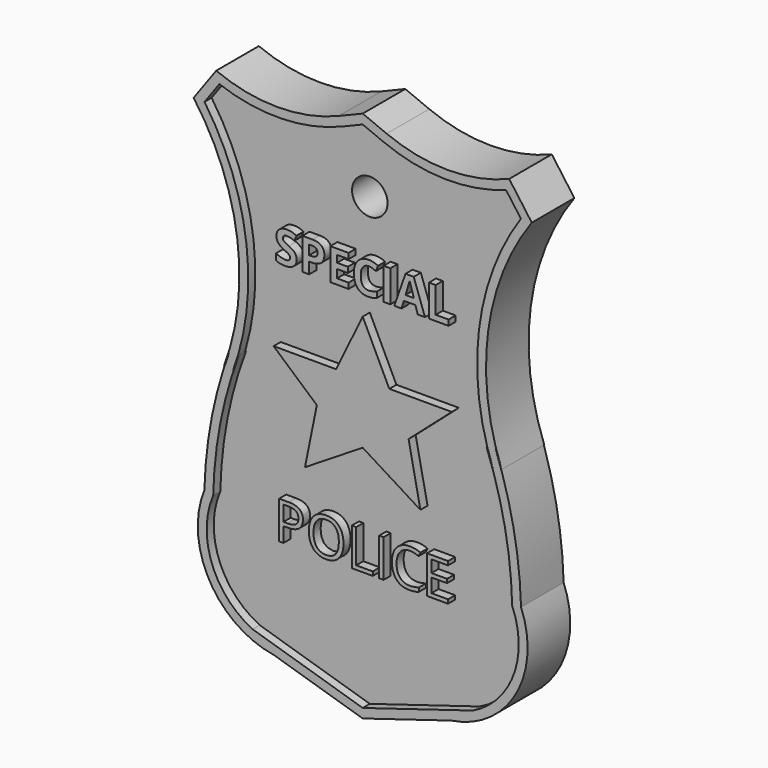
from build123d import *

# Parameters (mm, degrees)
F0_W           = 0.4923276621
F0_H           = 4.2362431042
F0_R           = 2
F0_W_2         = 0.7584236685
F0_H_2         = 3.5760967401
F1_DEPTH       = 5
F0_TEXT_SIZE   = 5.0091965718
F0_TEXT_SIZE_2 = 5.9338927263
F2_DEPTH       = 6


# Not quite as in the source:
# - a feature names something its author has since deleted; it is built from what else it names
# - Text() gives the source's letters only with a copy of the font that has no kerning and outlines rounded to 1/6400 em; it was checked with that copy


with BuildPart() as f1:
    # F0 (on Front) → F1 (new body)
    with BuildSketch(Plane.XZ):
        with BuildLine():
            Line((2.6978656745, 27.0723157725), (0, 28.1849289482))
            Line((0, 28.1849289482), (-2.6978656745, 27.0723157725))
            ThreePointArc((-2.6978656745, 27.0723157725), (-9.601713641, 25.7045974419), (-16.5055616074, 27.0723157725))
            Line((-16.5055616074, 27.0723157725), (-19.0506021551, 23.561483789))
            ThreePointArc((-19.0506021551, 23.561483789), (-14.1307840894, 11.1964219838), (-15.6559578137, -2.0237598742))
            Line((-15.6559578137, -2.0237598742), (-14.8904452178, 0))
            ThreePointArc((-14.8904452178, 0), (-16.9912920381, -7.3586022254), (-17.8392625093, -14.9640956448))
            ThreePointArc((-17.8392625093, -14.9640956448), (-17.2572372048, -23.7734712257), (-9.9838551694, -28.7776460174))
            Line((-9.9838551694, -28.7776460174), (0, -31.8150710518))
            Line((0, -31.8150710518), (9.9838551694, -28.7776460174))
            ThreePointArc((9.9838551694, -28.7776460174), (17.2572372048, -23.7734712257), (17.8392625093, -14.9640956448))
            ThreePointArc((17.8392625093, -14.9640956448), (16.9912920381, -7.3586022254), (14.8904452178, 0))
            Line((14.8904452178, 0), (15.6559578137, -2.0237598742))
            ThreePointArc((15.6559578137, -2.0237598742), (14.1307840894, 11.1964219838), (19.0506021551, 23.561483789))
            Line((19.0506021551, 23.561483789), (16.5055616074, 27.0723157725))
            ThreePointArc((16.5055616074, 27.0723157725), (9.601713641, 25.7045974419), (2.6978656745, 27.0723157725))
        make_face()
        with BuildLine():
            Line((-17.8220764571, 23.5524013394), (-16.1484710633, 25.8611061456))
            ThreePointArc((-16.1484710633, 25.8611061456), (-9.2056785313, 24.7087019846), (-2.3166098411, 26.1478462006))
            Line((-2.3166098411, 26.1478462006), (0, 27.1032275809))
            Line((0, 27.1032275809), (2.3166098411, 26.1478462006))
            ThreePointArc((2.3166098411, 26.1478462006), (9.2056785313, 24.7087019846), (16.1484710633, 25.8611061456))
            Line((16.1484710633, 25.8611061456), (17.8220764571, 23.5524013394))
            ThreePointArc((17.8220764571, 23.5524013394), (13.0939999284, 10.9674605371), (14.7206357065, -2.3775572112))
            Line((14.7206357065, -2.3775572112), (13.9551231106, -0.353797337))
            ThreePointArc((13.9551231106, -0.353797337), (16.0279163768, -7.642539104), (16.8443387914, -15.1761758693))
            ThreePointArc((16.8443387914, -15.1761758693), (16.9968634432, -21.9803415725), (12.3984711461, -26.9977834474))
            Line((12.3984711461, -26.9977834474), (0, -30.7698159948))
            Line((0, -30.7698159948), (-12.3984711461, -26.9977834474))
            ThreePointArc((-12.3984711461, -26.9977834474), (-16.9968634432, -21.9803415725), (-16.8443387914, -15.1761758693))
            ThreePointArc((-16.8443387914, -15.1761758693), (-16.0279163768, -7.642539104), (-13.9551231106, -0.353797337))
            Line((-13.9551231106, -0.353797337), (-14.7206357065, -2.3775572112))
            ThreePointArc((-14.7206357065, -2.3775572112), (-13.0939999284, 10.9674605371), (-17.8220764571, 23.5524013394))
        make_face(mode=Mode.SUBTRACT)
        with BuildLine():
            ThreePointArc((-2.3166098411, 26.1478462006), (-9.2056785313, 24.7087019846), (-16.1484710633, 25.8611061456))
            Line((-16.1484710633, 25.8611061456), (-17.8220764571, 23.5524013394))
            ThreePointArc((-17.8220764571, 23.5524013394), (-13.0939999284, 10.9674605371), (-14.7206357065, -2.3775572112))
            Line((-14.7206357065, -2.3775572112), (-13.9551231106, -0.353797337))
            ThreePointArc((-13.9551231106, -0.353797337), (-16.0279163768, -7.642539104), (-16.8443387914, -15.1761758693))
            ThreePointArc((-16.8443387914, -15.1761758693), (-16.9968634432, -21.9803415725), (-12.3984711461, -26.9977834474))
            Line((-12.3984711461, -26.9977834474), (0, -30.7698159948))
            Line((0, -30.7698159948), (12.3984711461, -26.9977834474))
            ThreePointArc((12.3984711461, -26.9977834474), (16.9968634432, -21.9803415725), (16.8443387914, -15.1761758693))
            ThreePointArc((16.8443387914, -15.1761758693), (16.0279163768, -7.642539104), (13.9551231106, -0.353797337))
            Line((13.9551231106, -0.353797337), (14.7206357065, -2.3775572112))
            ThreePointArc((14.7206357065, -2.3775572112), (13.0939999284, 10.9674605371), (17.8220764571, 23.5524013394))
            Line((17.8220764571, 23.5524013394), (16.1484710633, 25.8611061456))
            ThreePointArc((16.1484710633, 25.8611061456), (9.2056785313, 24.7087019846), (2.3166098411, 26.1478462006))
            Line((2.3166098411, 26.1478462006), (0, 27.1032275809))
            Line((0, 27.1032275809), (-2.3166098411, 26.1478462006))
        make_face()
        with BuildLine():
            add(Edge.make_bspline(
                [(-8.3190394511, -13.0703245643), (-6.7317231468, -13.0703245643), (-6.7317231468, -14.3043888173)],
                knots=[0, 0, 0, 1, 1, 1], degree=2))
            add(Edge.make_bspline(
                [(-6.7317231468, -14.3043888173), (-6.7317231468, -14.9478453098), (-7.1707384915, -15.2941435806)],
                knots=[0, 0, 0, 1, 1, 1], degree=2))
            add(Edge.make_bspline(
                [(-7.1707384915, -15.2941435806), (-7.6097538362, -15.6404418514), (-8.4265912568, -15.6404418514)],
                knots=[0, 0, 0, 1, 1, 1], degree=2))
            Line((-8.4265912568, -15.6404418514), (-8.9254091141, -15.6404418514))
            Line((-8.9254091141, -15.6404418514), (-8.9254091141, -17.3065676685))
            Line((-8.9254091141, -17.3065676685), (-9.4177367762, -17.3065676685))
            Line((-9.4177367762, -17.3065676685), (-9.4177367762, -13.0703245643))
            Line((-9.4177367762, -13.0703245643), (-8.3190394511, -13.0703245643))
        make_face(mode=Mode.SUBTRACT)
        with BuildLine():
            add(Edge.make_bspline(
                [(-2.6809141903, -13.5830499827), (-2.168188772, -14.1625316943), (-2.168188772, -15.1824195066)],
                knots=[0, 0, 0, 1, 1, 1], degree=2))
            add(Edge.make_bspline(
                [(-2.168188772, -15.1824195066), (-2.168188772, -16.1995258068), (-2.6827685318, -16.7822526159)],
                knots=[0, 0, 0, 1, 1, 1], degree=2))
            add(Edge.make_bspline(
                [(-2.6827685318, -16.7822526159), (-3.1973482917, -17.364979425), (-4.1124658106, -17.364979425)],
                knots=[0, 0, 0, 1, 1, 1], degree=2))
            add(Edge.make_bspline(
                [(-4.1124658106, -17.364979425), (-5.0479810857, -17.364979425), (-5.5565342358, -16.792451494)],
                knots=[0, 0, 0, 1, 1, 1], degree=2))
            add(Edge.make_bspline(
                [(-5.5565342358, -16.792451494), (-6.0650873858, -16.219923563), (-6.0650873858, -15.1768564822)],
                knots=[0, 0, 0, 1, 1, 1], degree=2))
            add(Edge.make_bspline(
                [(-6.0650873858, -15.1768564822), (-6.0650873858, -14.142133938), (-5.5551434797, -13.5728511046)],
                knots=[0, 0, 0, 1, 1, 1], degree=2))
            add(Edge.make_bspline(
                [(-5.5551434797, -13.5728511046), (-5.0451995735, -13.0035682712), (-4.1069027861, -13.0035682712)],
                knots=[0, 0, 0, 1, 1, 1], degree=2))
            add(Edge.make_bspline(
                [(-4.1069027861, -13.0035682712), (-3.1936396087, -13.0035682712), (-2.6809141903, -13.5830499827)],
                knots=[0, 0, 0, 1, 1, 1], degree=2))
        make_face(mode=Mode.SUBTRACT)
        Polygon((1.1371749108, -17.3065676685), (-1.2243289602, -17.3065676685), (-1.2243289602, -13.0703245643), (-0.732001298, -13.0703245643), (-0.732001298, -16.8605985433), (1.1371749108, -16.8605985433), align=None, mode=Mode.SUBTRACT)
        with Locations((2.1018960642, -15.1884461164)):
            Rectangle(F0_W, F0_H, mode=Mode.SUBTRACT)
        with BuildLine():
            add(Edge.make_bspline(
                [(6.2857540216, -13.6757670566), (5.8045524083, -13.4504645671), (5.323350795, -13.4504645671)],
                knots=[0, 0, 0, 1, 1, 1], degree=2))
            add(Edge.make_bspline(
                [(5.323350795, -13.4504645671), (4.625191229, -13.4504645671), (4.220944787, -13.9154406925)],
                knots=[0, 0, 0, 1, 1, 1], degree=2))
            add(Edge.make_bspline(
                [(4.220944787, -13.9154406925), (3.816698345, -14.3804168178), (3.816698345, -15.1889097018)],
                knots=[0, 0, 0, 1, 1, 1], degree=2))
            add(Edge.make_bspline(
                [(3.816698345, -15.1889097018), (3.816698345, -16.0196546835), (4.2065736405, -16.47350476)],
                knots=[0, 0, 0, 1, 1, 1], degree=2))
            add(Edge.make_bspline(
                [(4.2065736405, -16.47350476), (4.5964489361, -16.9273548365), (5.3177877706, -16.9273548365)],
                knots=[0, 0, 0, 1, 1, 1], degree=2))
            add(Edge.make_bspline(
                [(5.3177877706, -16.9273548365), (5.7609753836, -16.9273548365), (6.3293310463, -16.7678814695)],
                knots=[0, 0, 0, 1, 1, 1], degree=2))
            Line((6.3293310463, -16.7678814695), (6.3293310463, -17.1990158629))
            add(Edge.make_bspline(
                [(6.3293310463, -17.1990158629), (5.8889249455, -17.364979425), (5.2426869408, -17.364979425)],
                knots=[0, 0, 0, 1, 1, 1], degree=2))
            add(Edge.make_bspline(
                [(5.2426869408, -17.364979425), (4.3071716657, -17.364979425), (3.7986185156, -16.7966237623)],
                knots=[0, 0, 0, 1, 1, 1], degree=2))
            add(Edge.make_bspline(
                [(3.7986185156, -16.7966237623), (3.2900653655, -16.2282680997), (3.2900653655, -15.1824195066)],
                knots=[0, 0, 0, 1, 1, 1], degree=2))
            add(Edge.make_bspline(
                [(3.2900653655, -15.1824195066), (3.2900653655, -14.5278369653), (3.5348384405, -14.0355093031)],
                knots=[0, 0, 0, 1, 1, 1], degree=2))
            add(Edge.make_bspline(
                [(3.5348384405, -14.0355093031), (3.7796115155, -13.543181641), (4.2418061286, -13.2766200537)],
                knots=[0, 0, 0, 1, 1, 1], degree=2))
            add(Edge.make_bspline(
                [(4.2418061286, -13.2766200537), (4.7040007417, -13.0100584663), (5.3298409902, -13.0100584663)],
                knots=[0, 0, 0, 1, 1, 1], degree=2))
            add(Edge.make_bspline(
                [(5.3298409902, -13.0100584663), (5.9955495805, -13.0100584663), (6.4943674378, -13.2529771998)],
                knots=[0, 0, 0, 1, 1, 1], degree=2))
            Line((6.4943674378, -13.2529771998), (6.2857540216, -13.6757670566))
        make_face(mode=Mode.SUBTRACT)
        Polygon((9.6152241435, -16.8661615677), (9.6152241435, -17.3065676685), (7.2537202726, -17.3065676685), (7.2537202726, -13.0703245643), (9.6152241435, -13.0703245643), (9.6152241435, -13.5079491529), (7.7460479347, -13.5079491529), (7.7460479347, -14.87274448), (9.5021093134, -14.87274448), (9.5021093134, -15.3075875563), (7.7460479347, -15.3075875563), (7.7460479347, -16.8661615677), align=None, mode=Mode.SUBTRACT)
        Polygon((-2.9973116953, 1.8562454497), (0, 8.0466551414), (2.9973116953, 1.8562454497), (10.0362910237, 1.8562454497), (5.1685351705, -2.4151530963), (6.5026363504, -9.0073454569), (0, -4.953042775), (-6.5026363504, -9.0073454569), (-5.1685351705, -2.4151530963), (-10.0362910237, 1.8562454497), align=None, mode=Mode.SUBTRACT)
        with BuildLine():
            add(Edge.make_bspline(
                [(-7.6249364067, 11.858161132), (-7.4390482527, 11.6174848904), (-7.4390482527, 11.2676238174)],
                knots=[0, 0, 0, 1, 1, 1], degree=2))
            add(Edge.make_bspline(
                [(-7.4390482527, 11.2676238174), (-7.4390482527, 10.7831405864), (-7.7877352953, 10.5041126836)],
                knots=[0, 0, 0, 1, 1, 1], degree=2))
            add(Edge.make_bspline(
                [(-7.7877352953, 10.5041126836), (-8.1364223379, 10.2250847809), (-8.7570931006, 10.2250847809)],
                knots=[0, 0, 0, 1, 1, 1], degree=2))
            add(Edge.make_bspline(
                [(-8.7570931006, 10.2250847809), (-9.3300199585, 10.2250847809), (-9.7698900325, 10.441106383)],
                knots=[0, 0, 0, 1, 1, 1], degree=2))
            Line((-9.7698900325, 10.441106383), (-9.7698900325, 11.1455246509))
            add(Edge.make_bspline(
                [(-9.7698900325, 11.1455246509), (-9.408288655, 10.9835084493), (-9.1574374829, 10.9177627443)],
                knots=[0, 0, 0, 1, 1, 1], degree=2))
            add(Edge.make_bspline(
                [(-9.1574374829, 10.9177627443), (-8.9065863108, 10.8520170393), (-8.6983915783, 10.8520170393)],
                knots=[0, 0, 0, 1, 1, 1], degree=2))
            add(Edge.make_bspline(
                [(-8.6983915783, 10.8520170393), (-8.4494971236, 10.8520170393), (-8.3160489962, 10.9471135055)],
                knots=[0, 0, 0, 1, 1, 1], degree=2))
            add(Edge.make_bspline(
                [(-8.3160489962, 10.9471135055), (-8.1826008688, 11.0422099716), (-8.1826008688, 11.23083753)],
                knots=[0, 0, 0, 1, 1, 1], degree=2))
            add(Edge.make_bspline(
                [(-8.1826008688, 11.23083753), (-8.1826008688, 11.3357175833), (-8.2413023911, 11.4178997145)],
                knots=[0, 0, 0, 1, 1, 1], degree=2))
            add(Edge.make_bspline(
                [(-8.2413023911, 11.4178997145), (-8.3000039134, 11.5000818458), (-8.4138848667, 11.5756111378)],
                knots=[0, 0, 0, 1, 1, 1], degree=2))
            add(Edge.make_bspline(
                [(-8.4138848667, 11.5756111378), (-8.5277658201, 11.6511404299), (-8.8776268931, 11.8178527533)],
                knots=[0, 0, 0, 1, 1, 1], degree=2))
            add(Edge.make_bspline(
                [(-8.8776268931, 11.8178527533), (-9.2047900442, 11.9720420853), (-9.3687629633, 12.1137084258)],
                knots=[0, 0, 0, 1, 1, 1], degree=2))
            add(Edge.make_bspline(
                [(-9.3687629633, 12.1137084258), (-9.5327358823, 12.2553747664), (-9.6305717528, 12.4440023248)],
                knots=[0, 0, 0, 1, 1, 1], degree=2))
            add(Edge.make_bspline(
                [(-9.6305717528, 12.4440023248), (-9.7284076234, 12.6326298832), (-9.7284076234, 12.8838723987)],
                knots=[0, 0, 0, 1, 1, 1], degree=2))
            add(Edge.make_bspline(
                [(-9.7284076234, 12.8838723987), (-9.7284076234, 13.3589633861), (-9.406723281, 13.6301644192)],
                knots=[0, 0, 0, 1, 1, 1], degree=2))
            add(Edge.make_bspline(
                [(-9.406723281, 13.6301644192), (-9.0850389387, 13.9013654524), (-8.5175908895, 13.9013654524)],
                knots=[0, 0, 0, 1, 1, 1], degree=2))
            add(Edge.make_bspline(
                [(-8.5175908895, 13.9013654524), (-8.2389543302, 13.9013654524), (-7.9857550972, 13.8356197474)],
                knots=[0, 0, 0, 1, 1, 1], degree=2))
            add(Edge.make_bspline(
                [(-7.9857550972, 13.8356197474), (-7.7325558643, 13.7698740424), (-7.4562673659, 13.6501229368)],
                knots=[0, 0, 0, 1, 1, 1], degree=2))
            Line((-7.4562673659, 13.6501229368), (-7.7004656987, 13.0599769657))
            add(Edge.make_bspline(
                [(-7.7004656987, 13.0599769657), (-7.9869291277, 13.1773800104), (-8.1739913122, 13.2239498848)],
                knots=[0, 0, 0, 1, 1, 1], degree=2))
            add(Edge.make_bspline(
                [(-8.1739913122, 13.2239498848), (-8.3610534967, 13.2705197591), (-8.5418541854, 13.2705197591)],
                knots=[0, 0, 0, 1, 1, 1], degree=2))
            add(Edge.make_bspline(
                [(-8.5418541854, 13.2705197591), (-8.7570931006, 13.2705197591), (-8.8721480844, 13.1703358277)],
                knots=[0, 0, 0, 1, 1, 1], degree=2))
            add(Edge.make_bspline(
                [(-8.8721480844, 13.1703358277), (-8.9872030681, 13.0701518963), (-8.9872030681, 12.9089183816)],
                knots=[0, 0, 0, 1, 1, 1], degree=2))
            add(Edge.make_bspline(
                [(-8.9872030681, 12.9089183816), (-8.9872030681, 12.8087344502), (-8.9406331938, 12.7339878451)],
                knots=[0, 0, 0, 1, 1, 1], degree=2))
            add(Edge.make_bspline(
                [(-8.9406331938, 12.7339878451), (-8.8940633194, 12.65924124), (-8.7927053575, 12.5895821001)],
                knots=[0, 0, 0, 1, 1, 1], degree=2))
            add(Edge.make_bspline(
                [(-8.7927053575, 12.5895821001), (-8.6913473956, 12.5199229603), (-8.3125269049, 12.3391222716)],
                knots=[0, 0, 0, 1, 1, 1], degree=2))
            add(Edge.make_bspline(
                [(-8.3125269049, 12.3391222716), (-7.8108245607, 12.0988373735), (-7.6249364067, 11.858161132)],
                knots=[0, 0, 0, 1, 1, 1], degree=2))
        make_face(mode=Mode.SUBTRACT)
        with BuildLine():
            add(Edge.make_bspline(
                [(-4.6593354988, 13.5702888665), (-4.3208233867, 13.2900869332), (-4.3208233867, 12.7351618755)],
                knots=[0, 0, 0, 1, 1, 1], degree=2))
            add(Edge.make_bspline(
                [(-4.3208233867, 12.7351618755), (-4.3208233867, 12.1575388958), (-4.6816420773, 11.8518996362)],
                knots=[0, 0, 0, 1, 1, 1], degree=2))
            add(Edge.make_bspline(
                [(-4.6816420773, 11.8518996362), (-5.0424607678, 11.5462603767), (-5.7077446875, 11.5462603767)],
                knots=[0, 0, 0, 1, 1, 1], degree=2))
            Line((-5.7077446875, 11.5462603767), (-6.0325597777, 11.5462603767))
            Line((-6.0325597777, 11.5462603767), (-6.0325597777, 10.2743940596))
            Line((-6.0325597777, 10.2743940596), (-6.7909834462, 10.2743940596))
            Line((-6.7909834462, 10.2743940596), (-6.7909834462, 13.8504907997))
            Line((-6.7909834462, 13.8504907997), (-5.6490431652, 13.8504907997))
            add(Edge.make_bspline(
                [(-5.6490431652, 13.8504907997), (-4.9978476108, 13.8504907997), (-4.6593354988, 13.5702888665)],
                knots=[0, 0, 0, 1, 1, 1], degree=2))
        make_face(mode=Mode.SUBTRACT)
        Polygon((-1.5861151333, 10.9005436311), (-1.5861151333, 10.2743940596), (-3.6453645365, 10.2743940596), (-3.6453645365, 13.8504907997), (-1.5861151333, 13.8504907997), (-1.5861151333, 13.22903735), (-2.886940868, 13.22903735), (-2.886940868, 12.4440023248), (-1.6761241342, 12.4440023248), (-1.6761241342, 11.8225488751), (-2.886940868, 11.8225488751), (-2.886940868, 10.9005436311), align=None, mode=Mode.SUBTRACT)
        with Locations((0, 19.5384901017)):
            Circle(F0_R, mode=Mode.SUBTRACT)
        with BuildLine():
            add(Edge.make_bspline(
                [(1.0773686064, 13.1996865889), (0.8746526827, 13.2705197591), (0.6789809416, 13.2705197591)],
                knots=[0, 0, 0, 1, 1, 1], degree=2))
            add(Edge.make_bspline(
                [(0.6789809416, 13.2705197591), (0.2508511721, 13.2705197591), (0.0160450828, 12.9488354168)],
                knots=[0, 0, 0, 1, 1, 1], degree=2))
            add(Edge.make_bspline(
                [(0.0160450828, 12.9488354168), (-0.2187610065, 12.6271510744), (-0.2187610065, 12.0526588426)],
                knots=[0, 0, 0, 1, 1, 1], degree=2))
            add(Edge.make_bspline(
                [(-0.2187610065, 12.0526588426), (-0.2187610065, 10.8567131611), (0.6789809416, 10.8567131611)],
                knots=[0, 0, 0, 1, 1, 1], degree=2))
            add(Edge.make_bspline(
                [(0.6789809416, 10.8567131611), (1.0554533714, 10.8567131611), (1.590811255, 11.0445580325)],
                knots=[0, 0, 0, 1, 1, 1], degree=2))
            Line((1.590811255, 11.0445580325), (1.590811255, 10.4090162175))
            add(Edge.make_bspline(
                [(1.590811255, 10.4090162175), (1.1509411811, 10.2250847809), (0.6077564278, 10.2250847809)],
                knots=[0, 0, 0, 1, 1, 1], degree=2))
            add(Edge.make_bspline(
                [(0.6077564278, 10.2250847809), (-0.1725824756, 10.2250847809), (-0.5858411928, 10.6986103943)],
                knots=[0, 0, 0, 1, 1, 1], degree=2))
            add(Edge.make_bspline(
                [(-0.5858411928, 10.6986103943), (-0.99909991, 11.1721360077), (-0.99909991, 12.0573549644)],
                knots=[0, 0, 0, 1, 1, 1], degree=2))
            add(Edge.make_bspline(
                [(-0.99909991, 12.0573549644), (-0.99909991, 12.61541077), (-0.7959926427, 13.0349309829)],
                knots=[0, 0, 0, 1, 1, 1], degree=2))
            add(Edge.make_bspline(
                [(-0.7959926427, 13.0349309829), (-0.5928853755, 13.4544511958), (-0.2124995108, 13.6779083241)],
                knots=[0, 0, 0, 1, 1, 1], degree=2))
            add(Edge.make_bspline(
                [(-0.2124995108, 13.6779083241), (0.1678863539, 13.9013654524), (0.6789809416, 13.9013654524)],
                knots=[0, 0, 0, 1, 1, 1], degree=2))
            add(Edge.make_bspline(
                [(0.6789809416, 13.9013654524), (1.1994677729, 13.9013654524), (1.7254334129, 13.6501229368)],
                knots=[0, 0, 0, 1, 1, 1], degree=2))
            Line((1.7254334129, 13.6501229368), (1.48123508, 13.0333656089))
            add(Edge.make_bspline(
                [(1.48123508, 13.0333656089), (1.2800845302, 13.1288534186), (1.0773686064, 13.1996865889)],
                knots=[0, 0, 0, 1, 1, 1], degree=2))
        make_face(mode=Mode.SUBTRACT)
        with Locations((2.7307948186, 12.0624424297)):
            Rectangle(F0_W_2, F0_H_2, mode=Mode.SUBTRACT)
        Polygon((7.0163972919, 10.2743940596), (6.1992721011, 10.2743940596), (5.9402027159, 11.1259574768), (4.6362462333, 11.1259574768), (4.3771768481, 10.2743940596), (3.5600516573, 10.2743940596), (4.8225257308, 13.865361852), (5.7492270966, 13.865361852), align=None, mode=Mode.SUBTRACT)
        Polygon((9.6751849098, 10.2743940596), (7.4664422964, 10.2743940596), (7.4664422964, 13.8504907997), (8.2248659649, 13.8504907997), (8.2248659649, 10.9005436311), (9.6751849098, 10.9005436311), align=None, mode=Mode.SUBTRACT)
    extrude(amount=F1_DEPTH)

    # F0 (on Front) → F2 (join)
    with BuildSketch(Plane.XZ):
        with BuildLine():
            Line((2.6978656745, 27.0723157725), (0, 28.1849289482))
            Line((0, 28.1849289482), (-2.6978656745, 27.0723157725))
            ThreePointArc((-2.6978656745, 27.0723157725), (-9.601713641, 25.7045974419), (-16.5055616074, 27.0723157725))
            Line((-16.5055616074, 27.0723157725), (-19.0506021551, 23.561483789))
            ThreePointArc((-19.0506021551, 23.561483789), (-14.1307840894, 11.1964219838), (-15.6559578137, -2.0237598742))
            Line((-15.6559578137, -2.0237598742), (-14.8904452178, 0))
            ThreePointArc((-14.8904452178, 0), (-16.9912920381, -7.3586022254), (-17.8392625093, -14.9640956448))
            ThreePointArc((-17.8392625093, -14.9640956448), (-17.2572372048, -23.7734712257), (-9.9838551694, -28.7776460174))
            Line((-9.9838551694, -28.7776460174), (0, -31.8150710518))
            Line((0, -31.8150710518), (9.9838551694, -28.7776460174))
            ThreePointArc((9.9838551694, -28.7776460174), (17.2572372048, -23.7734712257), (17.8392625093, -14.9640956448))
            ThreePointArc((17.8392625093, -14.9640956448), (16.9912920381, -7.3586022254), (14.8904452178, 0))
            Line((14.8904452178, 0), (15.6559578137, -2.0237598742))
            ThreePointArc((15.6559578137, -2.0237598742), (14.1307840894, 11.1964219838), (19.0506021551, 23.561483789))
            Line((19.0506021551, 23.561483789), (16.5055616074, 27.0723157725))
            ThreePointArc((16.5055616074, 27.0723157725), (9.601713641, 25.7045974419), (2.6978656745, 27.0723157725))
        make_face()
        with BuildLine():
            Line((-17.8220764571, 23.5524013394), (-16.1484710633, 25.8611061456))
            ThreePointArc((-16.1484710633, 25.8611061456), (-9.2056785313, 24.7087019846), (-2.3166098411, 26.1478462006))
            Line((-2.3166098411, 26.1478462006), (0, 27.1032275809))
            Line((0, 27.1032275809), (2.3166098411, 26.1478462006))
            ThreePointArc((2.3166098411, 26.1478462006), (9.2056785313, 24.7087019846), (16.1484710633, 25.8611061456))
            Line((16.1484710633, 25.8611061456), (17.8220764571, 23.5524013394))
            ThreePointArc((17.8220764571, 23.5524013394), (13.0939999284, 10.9674605371), (14.7206357065, -2.3775572112))
            Line((14.7206357065, -2.3775572112), (13.9551231106, -0.353797337))
            ThreePointArc((13.9551231106, -0.353797337), (16.0279163768, -7.642539104), (16.8443387914, -15.1761758693))
            ThreePointArc((16.8443387914, -15.1761758693), (16.9968634432, -21.9803415725), (12.3984711461, -26.9977834474))
            Line((12.3984711461, -26.9977834474), (0, -30.7698159948))
            Line((0, -30.7698159948), (-12.3984711461, -26.9977834474))
            ThreePointArc((-12.3984711461, -26.9977834474), (-16.9968634432, -21.9803415725), (-16.8443387914, -15.1761758693))
            ThreePointArc((-16.8443387914, -15.1761758693), (-16.0279163768, -7.642539104), (-13.9551231106, -0.353797337))
            Line((-13.9551231106, -0.353797337), (-14.7206357065, -2.3775572112))
            ThreePointArc((-14.7206357065, -2.3775572112), (-13.0939999284, 10.9674605371), (-17.8220764571, 23.5524013394))
        make_face(mode=Mode.SUBTRACT)
        Polygon((2.9973116953, 1.8562454497), (0, 8.0466551414), (-2.9973116953, 1.8562454497), (-10.0362910237, 1.8562454497), (-5.1685351705, -2.4151530963), (-6.5026363504, -9.0073454569), (0, -4.953042775), (6.5026363504, -9.0073454569), (5.1685351705, -2.4151530963), (10.0362910237, 1.8562454497), align=None)
        with Locations((-10, 10.2743940596)):
            Text('SPECIAL', F0_TEXT_SIZE, font='Open Sans', font_style=FontStyle.BOLD, text_align=(TextAlign.LEFT, TextAlign.BOTTOM))
        with Locations((-10, -17.3065676685)):
            Text('POLICE', F0_TEXT_SIZE_2, font='Open Sans', text_align=(TextAlign.LEFT, TextAlign.BOTTOM))
    extrude(amount=F2_DEPTH)


with BuildPart() as f1b:
    # F0 (on Front) → F1, piece 2 (new body)
    with BuildSketch(Plane.XZ):
        with BuildLine():
            add(Edge.make_bspline(
                [(-5.1773214037, -13.8890163264), (-5.5440174308, -14.3340582809), (-5.5440174308, -15.1824195066)],
                knots=[0, 0, 0, 1, 1, 1], degree=2))
            add(Edge.make_bspline(
                [(-5.5440174308, -15.1824195066), (-5.5440174308, -16.042833952), (-5.1773214037, -16.4878759064)],
                knots=[0, 0, 0, 1, 1, 1], degree=2))
            add(Edge.make_bspline(
                [(-5.1773214037, -16.4878759064), (-4.8106253767, -16.9329178609), (-4.1124658106, -16.9329178609)],
                knots=[0, 0, 0, 1, 1, 1], degree=2))
            add(Edge.make_bspline(
                [(-4.1124658106, -16.9329178609), (-3.4087432201, -16.9329178609), (-3.0494645589, -16.4897302479)],
                knots=[0, 0, 0, 1, 1, 1], degree=2))
            add(Edge.make_bspline(
                [(-3.0494645589, -16.4897302479), (-2.6901858977, -16.0465426349), (-2.6901858977, -15.1824195066)],
                knots=[0, 0, 0, 1, 1, 1], degree=2))
            add(Edge.make_bspline(
                [(-2.6901858977, -15.1824195066), (-2.6901858977, -14.3275680857), (-3.0480738028, -13.8857712289)],
                knots=[0, 0, 0, 1, 1, 1], degree=2))
            add(Edge.make_bspline(
                [(-3.0480738028, -13.8857712289), (-3.4059617078, -13.443974372), (-4.1069027861, -13.443974372)],
                knots=[0, 0, 0, 1, 1, 1], degree=2))
            add(Edge.make_bspline(
                [(-4.1069027861, -13.443974372), (-4.8106253767, -13.443974372), (-5.1773214037, -13.8890163264)],
                knots=[0, 0, 0, 1, 1, 1], degree=2))
        make_face()
    extrude(amount=F1_DEPTH)


with BuildPart() as f1c:
    # F0 (on Front) → F1, piece 3 (new body)
    with BuildSketch(Plane.XZ):
        with BuildLine():
            Line((-8.9254091141, -13.4968231041), (-8.9254091141, -15.2176519947))
            Line((-8.9254091141, -15.2176519947), (-8.4812943304, -15.2176519947))
            add(Edge.make_bspline(
                [(-8.4812943304, -15.2176519947), (-7.826711789, -15.2176519947), (-7.534189421, -15.0062570663)],
                knots=[0, 0, 0, 1, 1, 1], degree=2))
            add(Edge.make_bspline(
                [(-7.534189421, -15.0062570663), (-7.241667053, -14.7948621379), (-7.241667053, -14.3275680857)],
                knots=[0, 0, 0, 1, 1, 1], degree=2))
            add(Edge.make_bspline(
                [(-7.241667053, -14.3275680857), (-7.241667053, -13.9075597412), (-7.5170367623, -13.7021914226)],
                knots=[0, 0, 0, 1, 1, 1], degree=2))
            add(Edge.make_bspline(
                [(-7.5170367623, -13.7021914226), (-7.7924064717, -13.4968231041), (-8.3746696954, -13.4968231041)],
                knots=[0, 0, 0, 1, 1, 1], degree=2))
            Line((-8.3746696954, -13.4968231041), (-8.9254091141, -13.4968231041))
        make_face()
    extrude(amount=F1_DEPTH)


with BuildPart() as f1d:
    # F0 (on Front) → F1, piece 4 (new body)
    with BuildSketch(Plane.XZ):
        with BuildLine():
            Line((-6.0325597777, 13.22903735), (-6.0325597777, 12.1677138264))
            Line((-6.0325597777, 12.1677138264), (-5.7828826361, 12.1677138264))
            add(Edge.make_bspline(
                [(-5.7828826361, 12.1677138264), (-5.43380425, 12.1677138264), (-5.2600477439, 12.3058580756)],
                knots=[0, 0, 0, 1, 1, 1], degree=2))
            add(Edge.make_bspline(
                [(-5.2600477439, 12.3058580756), (-5.0862912378, 12.4440023248), (-5.0862912378, 12.7077678318)],
                knots=[0, 0, 0, 1, 1, 1], degree=2))
            add(Edge.make_bspline(
                [(-5.0862912378, 12.7077678318), (-5.0862912378, 12.9746640866), (-5.2318710132, 13.1018507183)],
                knots=[0, 0, 0, 1, 1, 1], degree=2))
            add(Edge.make_bspline(
                [(-5.2318710132, 13.1018507183), (-5.3774507886, 13.22903735), (-5.6881775134, 13.22903735)],
                knots=[0, 0, 0, 1, 1, 1], degree=2))
            Line((-5.6881775134, 13.22903735), (-6.0325597777, 13.22903735))
        make_face()
    extrude(amount=F1_DEPTH)


with BuildPart() as f1e:
    # F0 (on Front) → F1, piece 5 (new body)
    with BuildSketch(Plane.XZ):
        with BuildLine():
            Line((4.8272218526, 11.7614992919), (5.7586193402, 11.7614992919))
            add(Edge.make_bspline(
                [(5.7586193402, 11.7614992919), (5.3993660236, 12.9183106252), (5.3539701796, 13.0701518963)],
                knots=[0, 0, 0, 1, 1, 1], degree=2))
            add(Edge.make_bspline(
                [(5.3539701796, 13.0701518963), (5.3085743357, 13.2219931673), (5.2890071616, 13.3096541073)],
                knots=[0, 0, 0, 1, 1, 1], degree=2))
            add(Edge.make_bspline(
                [(5.2890071616, 13.3096541073), (5.2083904043, 12.9965793216), (4.8272218526, 11.7614992919)],
                knots=[0, 0, 0, 1, 1, 1], degree=2))
        make_face()
    extrude(amount=F1_DEPTH)


solid = Compound([f1.part, f1b.part, f1c.part, f1d.part, f1e.part])
